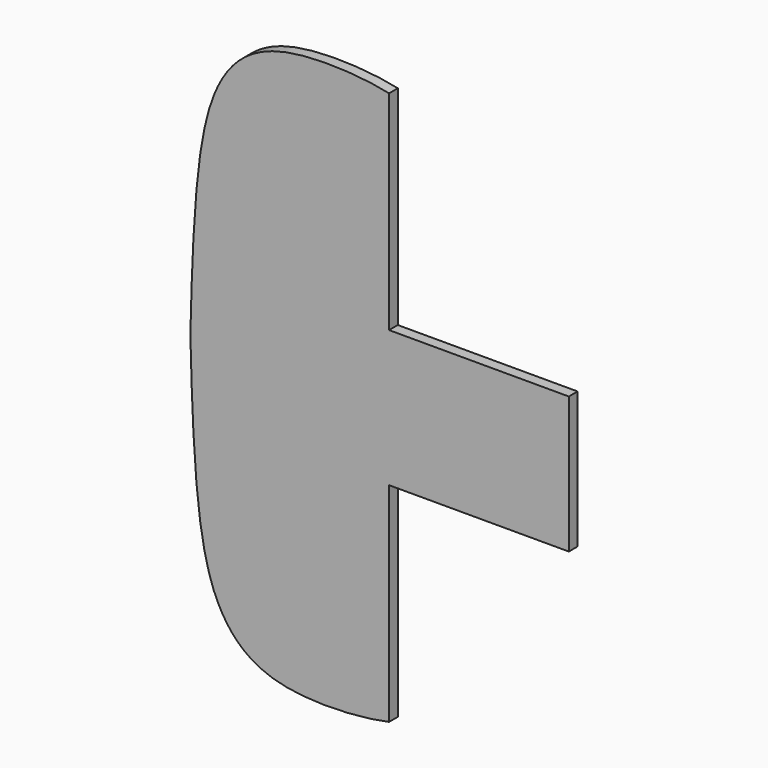
from build123d import *

# Parameters (mm, degrees)
F1_DEPTH    = 18
F2_T1_DEPTH = 30.2017817416


# Not quite as in the source:
# - a fillet or chamfer that OpenCascade refuses, or shapes differently, is made with other operations: its cross-section is extruded or revolved along the edge and cut away or added


with BuildPart() as f1:
    # F0 (on Front) → F1 (new body)
    with BuildSketch(Plane.XZ):
        with BuildLine():
            Line((295, -217), (-326, -217))
            add(Edge.make_bspline(
                [(0, -671), (-40.9557190503, -680.4161054833), (-182.3770697918, -691.4241372136), (-304.1643703394, -601.8547700973), (-320.5121159554, -444.292366147), (-326, -217)],
                knots=[0, 0, 0, 0, 0.3003903091, 0.5468271605, 1, 1, 1, 1], degree=3))
            Line((0, -671), (0, -329))
            Line((0, -329), (295, -329))
            Line((295, -329), (295, -217))
        make_face()
        with BuildLine():
            add(Edge.make_bspline(
                [(0, 237), (-40.9557190503, 246.4161054833), (-182.3770697918, 257.4241372136), (-304.1643703394, 167.8547700973), (-320.5121159554, 10.292366147), (-326, -217)],
                knots=[0, 0, 0, 0, 0.3003903091, 0.5468271605, 1, 1, 1, 1], degree=3))
            Line((-326, -217), (295, -217))
            Line((295, -217), (295, -105))
            Line((295, -105), (0, -105))
            Line((0, -105), (0, 237))
        make_face()
    extrude(amount=F1_DEPTH)

    # F2: fillet of radius 100 on 1 edges, made by hand

    # F2_s2 → F2_t1 (cut)
    with BuildSketch(Plane.XZ.offset(-6.1008908708)):
        with BuildLine():
            ThreePointArc((-325.941181539, -219.4396474121), (-325.9709446514, -217), (-325.941181539, -214.5603525879))
            Line((-325.941181539, -214.5603525879), (-335.9384452278, -214.3163878467))
            ThreePointArc((-335.9384452278, -214.3163878467), (-335.9677649192, -215.5375130178), (-335.9973263945, -216.7586185188))
            Line((-335.9973263945, -216.7586185188), (-335.9973263945, -217.2413814812))
            ThreePointArc((-335.9973263945, -217.2413814812), (-335.9677649192, -218.4624869822), (-335.9384452278, -219.6836121533))
            Line((-335.9384452278, -219.6836121533), (-325.941181539, -219.4396474121))
        make_face()
    extrude(amount=F2_T1_DEPTH, mode=Mode.SUBTRACT)


solid = f1.part
